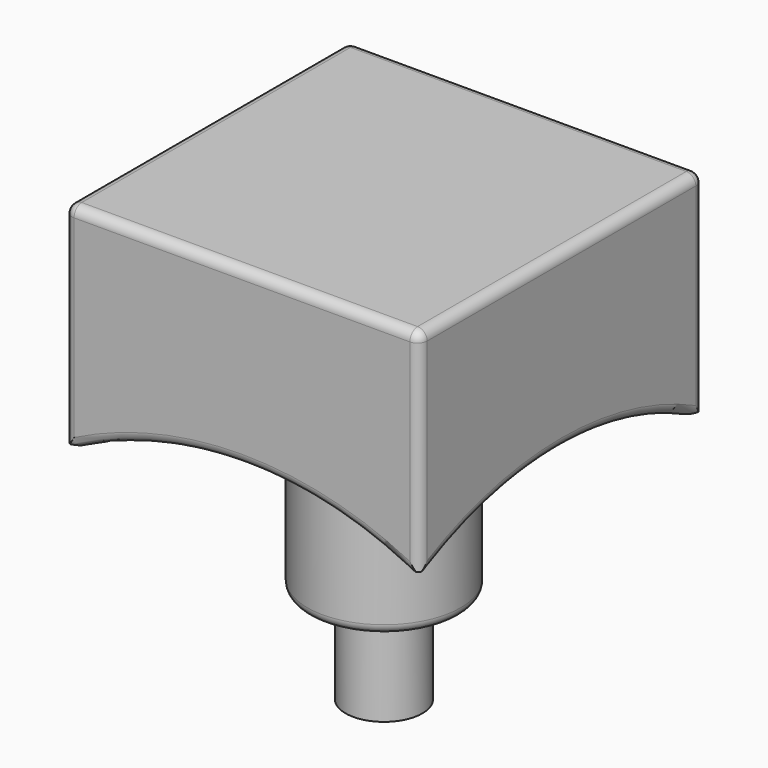
from build123d import *

# Parameters (mm, degrees)
F0_W          = 18.5
F0_H          = 11
F1_DEPTH      = 9.25
F2_DEPTH      = 9.25
F3_R          = 19
F5_DEPTH      = 25.4
F6_DEPTH      = 25.4
F4_R          = 19
F7_DEPTH      = 25.4
F8_DEPTH      = 25.4
F9_R          = 4
F10_DEPTH     = 3.45753
F11_DEPTH     = 7.5
F12_T1_DEPTH  = 11.75
F12_T3_DEPTH  = 17.5
F12_T5_DEPTH  = 17.5
F12_S9_W      = 0.5
F12_S9_H      = 0.5
F12_T10_DEPTH = 0.5
F12_S15_W     = 0.5
F12_S15_H     = 0.5
F12_T16_DEPTH = 0.5
F12_S21_W     = 0.5
F12_S21_H     = 0.5
F12_T22_DEPTH = 0.5
F12_S27_W     = 0.5
F12_S27_H     = 0.5
F12_T28_DEPTH = 0.5
F12_T34_ANGLE = 60.5906744424
F12_T36_ANGLE = 60.5906744424
F12_T38_ANGLE = 60.5906744424
F12_T40_ANGLE = 60.5906744424
F13_R         = 1.9993297739
F14_DEPTH     = 5


# Not quite as in the source:
# - a fillet or chamfer that OpenCascade refuses, or shapes differently, is made with other operations: its cross-section is extruded or revolved along the edge and cut away or added
# - a feature names something its author has since deleted; it is built from what else it names


with BuildPart() as f1:
    # F0 (on Front) → F1 (new body)
    with BuildSketch(Plane.XZ):
        Rectangle(F0_W, F0_H)
    extrude(amount=-F1_DEPTH)

    # F0 (on Front) → F2 (join)
    with BuildSketch(Plane.XZ):
        Rectangle(F0_W, F0_H)
    extrude(amount=F2_DEPTH)

    # F3 (on Front) → F5 (cut)
    with BuildSketch(Plane.XZ):
        with Locations((0, -22.5)):
            Circle(F3_R)
    extrude(amount=-F5_DEPTH, mode=Mode.SUBTRACT)

    # F3 (on Front) → F6 (cut)
    with BuildSketch(Plane.XZ):
        with Locations((0, -22.5)):
            Circle(F3_R)
    extrude(amount=F6_DEPTH, mode=Mode.SUBTRACT)

    # F4 (on Right) → F7 (cut)
    with BuildSketch(Plane.YZ):
        with Locations((0, -22.5)):
            Circle(F4_R)
    extrude(amount=-F7_DEPTH, mode=Mode.SUBTRACT)

    # F4 (on Right) → F8 (cut)
    with BuildSketch(Plane.YZ):
        with Locations((0, -22.5)):
            Circle(F4_R)
    extrude(amount=F8_DEPTH, mode=Mode.SUBTRACT)

    # F9 (on face) → F10 (join)
    with BuildSketch(Plane(origin=(0, 0, -5.5), x_dir=(1, 0, 0), z_dir=(0, 0, -1))):
        Circle(F9_R)
    extrude(amount=-F10_DEPTH)

    # F11 (add): a face of the model
    f11_faces = [f1.faces().sort_by_distance(p)[0] for p in [
        (0, 0, -5.5),
    ]]
    extrude(f11_faces, amount=F11_DEPTH)

    # F12: fillet of radius 0.5 on 13 edges, made by hand

    # F12_s2 → F12_t1 (cut)
    with BuildSketch(Plane.XY.offset(-6.75)):
        with BuildLine():
            ThreePointArc((9.25, -8.75), (9.1035533906, -9.1035533906), (8.75, -9.25))
            Line((8.75, -9.25), (9.25, -9.25))
            Line((9.25, -9.25), (9.25, -8.75))
        make_face()
        with BuildLine():
            ThreePointArc((-9.25, -8.75), (-9.1035533906, -9.1035533906), (-8.75, -9.25))
            Line((-8.75, -9.25), (-9.25, -9.25))
            Line((-9.25, -9.25), (-9.25, -8.75))
        make_face()
        with BuildLine():
            ThreePointArc((9.25, 8.75), (9.1035533906, 9.1035533906), (8.75, 9.25))
            Line((8.75, 9.25), (9.25, 9.25))
            Line((9.25, 9.25), (9.25, 8.75))
        make_face()
        with BuildLine():
            ThreePointArc((-8.75, 9.25), (-9.1035533906, 9.1035533906), (-9.25, 8.75))
            Line((-9.25, 8.75), (-9.25, 9.25))
            Line((-9.25, 9.25), (-8.75, 9.25))
        make_face()
    extrude(amount=F12_T1_DEPTH, mode=Mode.SUBTRACT)

    # F12_s4 → F12_t3 (cut)
    with BuildSketch(Plane.YZ.offset(-8.75)):
        with BuildLine():
            ThreePointArc((-8.75, 5.5), (-9.1035533906, 5.3535533906), (-9.25, 5))
            Line((-9.25, 5), (-9.25, 5.5))
            Line((-9.25, 5.5), (-8.75, 5.5))
        make_face()
        with BuildLine():
            ThreePointArc((9.25, 5), (9.1035533906, 5.3535533906), (8.75, 5.5))
            Line((8.75, 5.5), (9.25, 5.5))
            Line((9.25, 5.5), (9.25, 5))
        make_face()
    extrude(amount=F12_T3_DEPTH, mode=Mode.SUBTRACT)

    # F12_s6 → F12_t5 (cut)
    with BuildSketch(Plane.XZ.offset(-8.75)):
        with BuildLine():
            ThreePointArc((9.25, 5), (9.1035533906, 5.3535533906), (8.75, 5.5))
            Line((8.75, 5.5), (9.25, 5.5))
            Line((9.25, 5.5), (9.25, 5))
        make_face()
        with BuildLine():
            ThreePointArc((-9.25, 5), (-9.1035533906, 5.3535533906), (-8.75, 5.5))
            Line((-8.75, 5.5), (-9.25, 5.5))
            Line((-9.25, 5.5), (-9.25, 5))
        make_face()
    extrude(amount=F12_T5_DEPTH, mode=Mode.SUBTRACT)


with BuildPart() as f12_tool8:
    # F12_s9 → F12_t10 (new body)
    with BuildSketch(Plane.YZ.offset(8.75)):
        with Locations((-9, 5.25)):
            Rectangle(F12_S9_W, F12_S9_H)
    extrude(amount=F12_T10_DEPTH)

    # F12_s11 → F12_t12 (revolve, cut)
    with BuildSketch(Plane(origin=(8.75, -8.75, 5), x_dir=(0, 0.7071067812, -0.7071067812), z_dir=(0, -0.7071067812, -0.7071067812))):
        with BuildLine():
            ThreePointArc((0, -0.5), (0.5, 0), (0, 0.5))
            Line((0, 0.5), (0, -0.5))
        make_face()
    revolve(axis=Axis((8.75, -8.75, 5), (1, 0, 0)), mode=Mode.SUBTRACT)


with BuildPart() as f1_1:
    add(f1.part)

    # F12_t7: cut F12_tool8
    add(f12_tool8.part, mode=Mode.SUBTRACT)


with BuildPart() as f12_tool14:
    # F12_s15 → F12_t16 (new body)
    with BuildSketch(Plane.YZ.offset(-8.75)):
        with Locations((-9, 5.25)):
            Rectangle(F12_S15_W, F12_S15_H)
    extrude(amount=-F12_T16_DEPTH)

    # F12_s17 → F12_t18 (revolve, cut)
    with BuildSketch(Plane(origin=(-8.75, -8.75, 5), x_dir=(0, 0.7071067812, -0.7071067812), z_dir=(0, 0.7071067812, 0.7071067812))):
        with BuildLine():
            ThreePointArc((0, -0.5), (0.5, 0), (0, 0.5))
            Line((0, 0.5), (0, -0.5))
        make_face()
    revolve(axis=Axis((-8.75, -8.75, 5), (-1, 0, 0)), mode=Mode.SUBTRACT)


with BuildPart() as f1_2:
    add(f1_1.part)

    # F12_t13: cut F12_tool14
    add(f12_tool14.part, mode=Mode.SUBTRACT)


with BuildPart() as f12_tool20:
    # F12_s21 → F12_t22 (new body)
    with BuildSketch(Plane.YZ.offset(8.75)):
        with Locations((9, 5.25)):
            Rectangle(F12_S21_W, F12_S21_H)
    extrude(amount=F12_T22_DEPTH)

    # F12_s23 → F12_t24 (revolve, cut)
    with BuildSketch(Plane(origin=(8.75, 8.75, 5), x_dir=(0, -0.7071067812, -0.7071067812), z_dir=(0, -0.7071067812, 0.7071067812))):
        with BuildLine():
            ThreePointArc((0, -0.5), (0.5, 0), (0, 0.5))
            Line((0, 0.5), (0, -0.5))
        make_face()
    revolve(axis=Axis((8.75, 8.75, 5), (1, 0, 0)), mode=Mode.SUBTRACT)


with BuildPart() as f1_3:
    add(f1_2.part)

    # F12_t19: cut F12_tool20
    add(f12_tool20.part, mode=Mode.SUBTRACT)


with BuildPart() as f12_tool26:
    # F12_s27 → F12_t28 (new body)
    with BuildSketch(Plane.XZ.offset(-8.75)):
        with Locations((-9, 5.25)):
            Rectangle(F12_S27_W, F12_S27_H)
    extrude(amount=-F12_T28_DEPTH)

    # F12_s29 → F12_t30 (revolve, cut)
    with BuildSketch(Plane(origin=(-8.75, 8.75, 5), x_dir=(0.7071067812, 0, -0.7071067812), z_dir=(0.7071067812, 0, 0.7071067812))):
        with BuildLine():
            ThreePointArc((0, -0.5), (0.5, 0), (0, 0.5))
            Line((0, 0.5), (0, -0.5))
        make_face()
    revolve(axis=Axis((-8.75, 8.75, 5), (0, 1, 0)), mode=Mode.SUBTRACT)


with BuildPart() as f1_4:
    add(f1_3.part)

    # F12_t25: cut F12_tool26
    add(f12_tool26.part, mode=Mode.SUBTRACT)

    # F12_s31 → F12_t32 (revolve, cut)
    with BuildSketch(Plane.XZ):
        with BuildLine():
            ThreePointArc((4, -12.5), (3.8535533906, -12.8535533906), (3.5, -13))
            Line((3.5, -13), (4, -13))
            Line((4, -13), (4, -12.5))
        make_face()
    revolve(axis=Axis((0, 0, -13), (0, 0, -1)), mode=Mode.SUBTRACT)

    # F12_s33 → F12_t34 (revolve, cut)
    with BuildSketch(Plane(origin=(-9.8002563667, 0, -5.7257375924), x_dir=(0, 1, 0), z_dir=(-0.8634366066, 0, -0.5044573583))):
        with BuildLine():
            ThreePointArc((-8.75, 0.4273236492), (-9.1035533906, 0.2808770398), (-9.25, -0.0726763508))
            Line((-9.25, -0.0726763508), (-9.25, 0.4273236492))
            Line((-9.25, 0.4273236492), (-8.75, 0.4273236492))
        make_face()
    revolve(axis=Axis((0, -9.25, -22.5), (0, 1, 0)), revolution_arc=F12_T34_ANGLE, mode=Mode.SUBTRACT)

    # F12_s35 → F12_t36 (revolve, cut)
    with BuildSketch(Plane(origin=(0, 9.8002563667, -5.7257375924), x_dir=(1, 0, 0), z_dir=(0, 0.8634366066, -0.5044573583))):
        with BuildLine():
            ThreePointArc((-9.25, -0.0726763508), (-9.1035533906, 0.2808770398), (-8.75, 0.4273236492))
            Line((-8.75, 0.4273236492), (-9.25, 0.4273236492))
            Line((-9.25, 0.4273236492), (-9.25, -0.0726763508))
        make_face()
    revolve(axis=Axis((-9.25, 0, -22.5), (1, 0, 0)), revolution_arc=F12_T36_ANGLE, mode=Mode.SUBTRACT)

    # F12_s37 → F12_t38 (revolve, cut)
    with BuildSketch(Plane(origin=(0, -9.8002563667, -5.7257375924), x_dir=(1, 0, 0), z_dir=(0, -0.8634366066, -0.5044573583))):
        with BuildLine():
            ThreePointArc((9.25, 0.0726763508), (9.1035533906, -0.2808770398), (8.75, -0.4273236492))
            Line((8.75, -0.4273236492), (9.25, -0.4273236492))
            Line((9.25, -0.4273236492), (9.25, 0.0726763508))
        make_face()
    revolve(axis=Axis((9.25, 0, -22.5), (-1, 0, 0)), revolution_arc=F12_T38_ANGLE, mode=Mode.SUBTRACT)

    # F12_s39 → F12_t40 (revolve, cut)
    with BuildSketch(Plane(origin=(9.8002563667, 0, -5.7257375924), x_dir=(0, 1, 0), z_dir=(0.8634366066, 0, -0.5044573583))):
        with BuildLine():
            ThreePointArc((9.25, 0.0726763508), (9.1035533906, -0.2808770398), (8.75, -0.4273236492))
            Line((8.75, -0.4273236492), (9.25, -0.4273236492))
            Line((9.25, -0.4273236492), (9.25, 0.0726763508))
        make_face()
    revolve(axis=Axis((0, 9.25, -22.5), (0, -1, 0)), revolution_arc=F12_T40_ANGLE, mode=Mode.SUBTRACT)

    # F13 (on face) → F14 (join)
    with BuildSketch(Plane(origin=(0, 0, -13), x_dir=(1, 0, 0), z_dir=(0, 0, -1))):
        Circle(F13_R)
    extrude(amount=F14_DEPTH)


solid = f1_4.part
